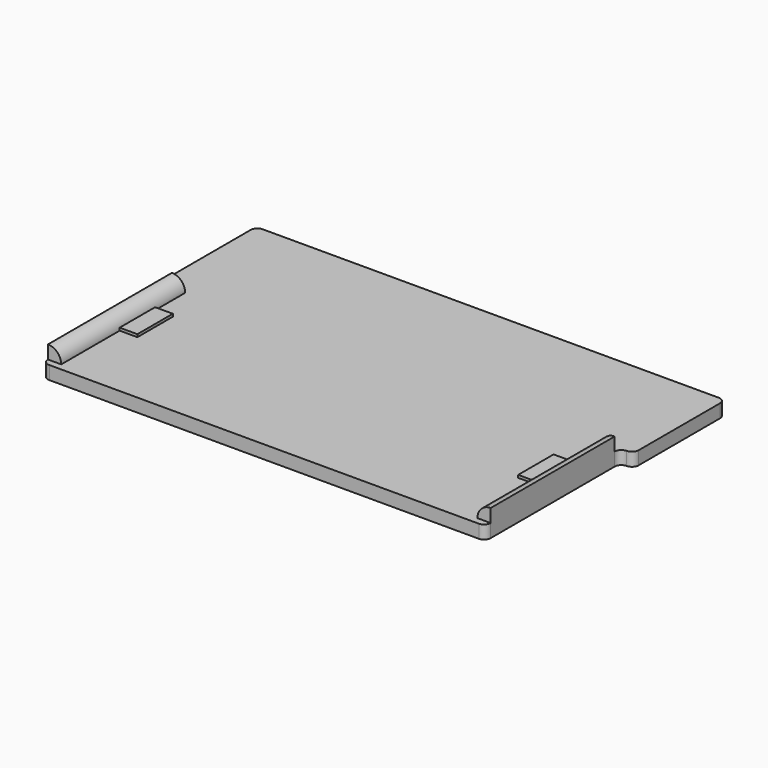
from build123d import *

# Parameters (mm, degrees)
F0_W     = 50
F0_H     = 19
F0_H_2   = 13
F0_W_2   = 1.5
F1_DEPTH = 1.5
F2_R     = 0.74999
F4_DEPTH = 1.5
F5_R     = 1.49999
F3_W     = 2
F3_H     = 5
F6_DEPTH = 0.3


# Not quite as in the source:
# - a fillet or chamfer is up to 0.001 mm smaller than in the source, because OpenCascade refuses the exact size


with BuildPart() as f1:
    # F0 (on Top) → F1 (new body)
    with BuildSketch(Plane.XY):
        with Locations((0, -6.5)):
            Rectangle(F0_W, F0_H)
        with Locations((0, 9.5)):
            Rectangle(F0_W, F0_H_2)
        with Locations((-25.75, 9.5)):
            Rectangle(F0_W_2, F0_H_2)
        with Locations((25.75, 9.5)):
            Rectangle(F0_W_2, F0_H_2)
    extrude(amount=F1_DEPTH)

    # F2 (radius 0.75 in the source; OpenCascade refuses exactly that, so slightly less here)
    f2_edges = [f1.edges().sort_by_distance(p)[0] for p in [
        (-26.5, 16, 0.75),
        (-26.5, 3, 0.75),
        (-25, 3, 0.75),
        (-25, -16, 0.75),
        (25, -16, 0.75),
        (25, 3, 0.75),
        (26.5, 3, 0.75),
        (26.5, 16, 0.75),
    ]]
    fillet(f2_edges, radius=F2_R)

    # F3 (on face) → F4 (join)
    with BuildSketch(Plane.XY.offset(1.5)):
        Polygon((-23.5, 2.25), (-25, 2.25), (-25, -15.25), (-23.5, -15.25), (-23.5, -7), (-23.5, -2), align=None)
        Polygon((23.5, -15.25), (25, -15.25), (25, 2.25), (23.5, 2.25), (23.5, -2), (23.5, -7), align=None)
    extrude(amount=F4_DEPTH)

    # F5 (radius 1.5 in the source; OpenCascade refuses exactly that, so slightly less here)
    f5_edges = [f1.edges().sort_by_distance(p)[0] for p in [
        (-23.5, -6.5, 3),
        (23.5, -6.5, 3),
    ]]
    fillet(f5_edges, radius=F5_R)

    # F3 (on face) → F6 (join)
    with BuildSketch(Plane.XY.offset(1.5)):
        with Locations((-22.5, -4.5)):
            Rectangle(F3_W, F3_H)
        with Locations((22.5, -4.5)):
            Rectangle(F3_W, F3_H)
    extrude(amount=F6_DEPTH)


solid = f1.part
